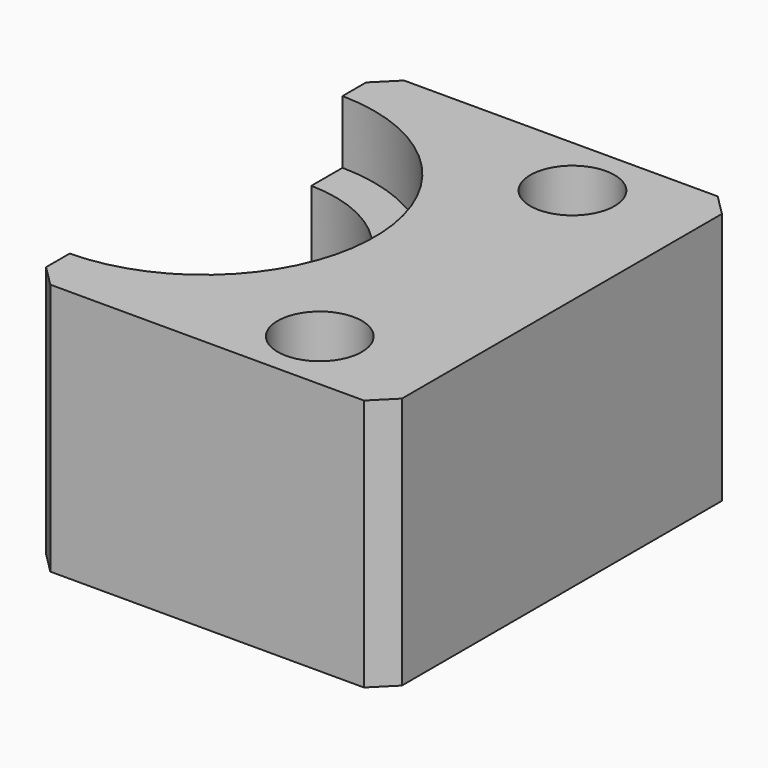
from build123d import *

# Parameters (mm, degrees)
F0_R     = 2
F1_DEPTH = 12
F2_R     = 8.1
F3_DEPTH = 3
F4_R     = 6.25
F5_DEPTH = 5.5
F6_R     = 8.1
F7_DEPTH = 25
F8_SIZE  = 1


with BuildPart() as f1:
    # F0 (on Top) → F1 (new body)
    with BuildSketch(Plane.XY):
        with BuildLine():
            Line((-0.9, -10.5), (16, -10.5))
            Line((16, -10.5), (16, 10.5))
            Line((16, 10.5), (-0.9, 10.5))
            Line((-0.9, 10.5), (-0.9, 0.9949874371))
            ThreePointArc((-0.9, 0.9949874371), (0, 0), (-0.9, -0.9949874371))
            Line((-0.9, -0.9949874371), (-0.9, -10.5))
        make_face()
        with Locations((10.5, -7.5)):
            Circle(F0_R, mode=Mode.SUBTRACT)
        with Locations((10.5, 7.5)):
            Circle(F0_R, mode=Mode.SUBTRACT)
    extrude(amount=F1_DEPTH)

    # F2 (on face) → F3 (cut)
    with BuildSketch(Plane.XY.offset(12)):
        with Locations((-1, 0)):
            Circle(F2_R)
    extrude(amount=-F3_DEPTH, mode=Mode.SUBTRACT)

    # F4 (on face) → F5 (cut)
    with BuildSketch(Plane.XY.offset(9)):
        with Locations((-1, 0)):
            Circle(F4_R)
    extrude(amount=-F5_DEPTH, mode=Mode.SUBTRACT)

    # F6 (on face) → F7 (cut)
    with BuildSketch(Plane.XY.offset(3.5)):
        with Locations((-1, 0)):
            Circle(F6_R)
    extrude(amount=-F7_DEPTH, mode=Mode.SUBTRACT)

    # F8
    f8_edges = [f1.edges().sort_by_distance(p)[0] for p in [
        (16, 10.5, 6),
        (16, -10.5, 6),
        (-0.9, -10.5, 6),
        (-0.9, 10.5, 6),
    ]]
    chamfer(f8_edges, length=F8_SIZE)


solid = f1.part
